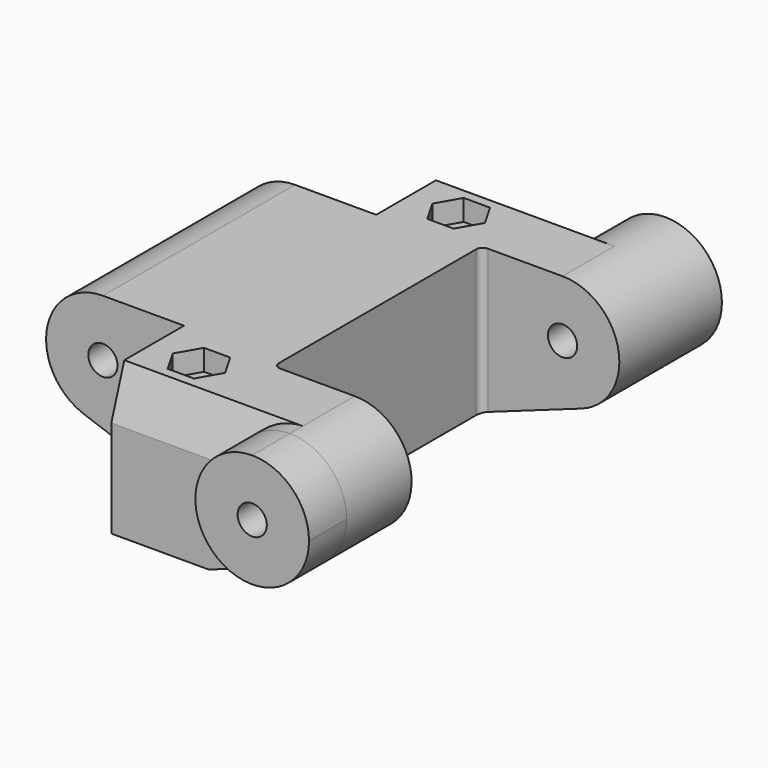
from build123d import *

# Parameters (mm, degrees)
F0_R          = 4.5
F1_DEPTH      = 65
F2_W          = 24.1539999843
F2_H          = 28
F2_W_2        = 25
F2_W_3        = 30
F2_H_2        = 80
F3_DEPTH      = 45.001
F4_R          = 4.5
F5_DEPTH      = 45.001
F6_R          = 4.5
F7_DEPTH      = 6.5
F8_R          = 4.5
F9_DEPTH      = 14.5
F10_T4_DEPTH  = 132.8518303197
F10_S5_R      = 17.5
F10_T6_DEPTH  = 68
F10_T10_DEPTH = 132.8518303197
F10_S11_R     = 17.5
F10_T12_DEPTH = 68
F11_R         = 2


# Not quite as in the source:
# - a fillet or chamfer that OpenCascade refuses, or shapes differently, is made with other operations: its cross-section is extruded or revolved along the edge and cut away or added
# - a pattern or mirror of a feature is missing from the dataset's text; its kind, count and spacing are read off the source's solid


with BuildPart() as f1:
    # F0 (on Front) → F1 (new body, symmetric)
    with BuildSketch(Plane.XZ):
        with BuildLine():
            Line((80, 17.5), (0, 17.5))
            ThreePointArc((0, 17.5), (-17.2437155554, 2.9840029898), (-5.880605574, -16.4823687036))
            Line((-5.880605574, -16.4823687036), (25, -27.5))
            Line((25, -27.5), (55, -27.5))
            Line((55, -27.5), (85.880605574, -16.4823687036))
            ThreePointArc((85.880605574, -16.4823687036), (97.2437155554, 2.9840029898), (80, 17.5))
        make_face()
        Circle(F0_R, mode=Mode.SUBTRACT)
        with Locations((80, 0)):
            Circle(F0_R, mode=Mode.SUBTRACT)
    extrude(amount=F1_DEPTH, both=True)

    # F2 (on face) → F3 (cut, through all)
    with BuildSketch(Plane.XY.offset(17.5)):
        with Locations((-12.0769999921, 51)):
            Rectangle(F2_W, F2_H)
        with Locations((12.5, 51)):
            Rectangle(F2_W_2, F2_H)
        with Locations((-12.0769999921, -51)):
            Rectangle(F2_W, F2_H)
        with Locations((12.5, -51)):
            Rectangle(F2_W_2, F2_H)
        Polygon((55, 40), (55, 0), (55, -40), (80, -40), (80, 40), align=None)
        with Locations((95, 0)):
            Rectangle(F2_W_3, F2_H_2)
    extrude(amount=-F3_DEPTH, mode=Mode.SUBTRACT)

    # F4 (on face) → F5 (cut, through all)
    with BuildSketch(Plane(origin=(0, 0, -27.5), x_dir=(1, 0, 0), z_dir=(0, 0, -1))):
        with Locations((40, 50)):
            Circle(F4_R)
        with Locations((40, -50)):
            Circle(F4_R)
    extrude(amount=-F5_DEPTH, mode=Mode.SUBTRACT)

    # F6 (on face) → F7 (cut)
    with BuildSketch(Plane.XY.offset(17.5)):
        Polygon((35.9585481157, 43), (44.0414518843, 43), (48.0829037687, 50), (44.0414518843, 57), (35.9585481157, 57), (31.9170962313, 50), align=None)
        with Locations((40, 50)):
            Circle(F6_R, mode=Mode.SUBTRACT)
        Polygon((44.0414518843, -57), (48.0829037687, -50), (44.0414518843, -43), (35.9585481157, -43), (31.9170962313, -50), (35.9585481157, -57), align=None)
        with Locations((40, -50)):
            Circle(F6_R, mode=Mode.SUBTRACT)
    extrude(amount=-F7_DEPTH, mode=Mode.SUBTRACT)

    # F8 (on face) → F9 (join)
    with BuildSketch(Plane.XZ.offset(65)):
        with BuildLine():
            ThreePointArc((85.880605574, -16.4823687036), (94.3031569513, -10.0831394529), (97.5, 0))
            ThreePointArc((97.5, 0), (92.3743686708, 12.3743686708), (80, 17.5))
            ThreePointArc((80, 17.5), (62.7562844446, -2.9840029898), (85.880605574, -16.4823687036))
        make_face()
        with Locations((80, 0)):
            Circle(F8_R, mode=Mode.SUBTRACT)
    f9 = extrude(amount=F9_DEPTH)

    # F9_copies: F9 across plane
    add(f9.mirror(Plane.ZX))

    # F10: chamfer of 5 x 15 on 2 edges, made by hand


with BuildPart() as f10_tool2:
    # F10_s3 → F10_t4 (new body)
    with BuildSketch(Plane.YZ.offset(118.9259151598)):
        Polygon((-60, 17.5), (-65, 2.5), (-65, 17.5), align=None)
    extrude(amount=-F10_T4_DEPTH)

    # F10_s5 → F10_t6 (cut, symmetric)
    with BuildSketch(Plane.XZ.offset(62.5)):
        with Locations((80, 0)):
            Circle(F10_S5_R)
    extrude(amount=F10_T6_DEPTH, both=True, mode=Mode.SUBTRACT)


with BuildPart() as f1_1:
    add(f1.part)

    # F10_t1: cut F10_tool2
    add(f10_tool2.part, mode=Mode.SUBTRACT)


with BuildPart() as f10_tool8:
    # F10_s9 → F10_t10 (new body)
    with BuildSketch(Plane.YZ.offset(118.9259151598)):
        Polygon((60, 17.5), (65, 2.5), (65, 17.5), align=None)
    extrude(amount=-F10_T10_DEPTH)

    # F10_s11 → F10_t12 (cut, symmetric)
    with BuildSketch(Plane.XZ.offset(-62.5)):
        with Locations((80, 0)):
            Circle(F10_S11_R)
    extrude(amount=F10_T12_DEPTH, both=True, mode=Mode.SUBTRACT)


with BuildPart() as f1_2:
    add(f1_1.part)

    # F10_t7: cut F10_tool8
    add(f10_tool8.part, mode=Mode.SUBTRACT)

    # F11
    f11_edges = [f1_2.edges().sort_by_distance(p)[0] for p in [
        (55, -40, -5),
        (55, 40, -5),
    ]]
    fillet(f11_edges, radius=F11_R)


solid = f1_2.part
